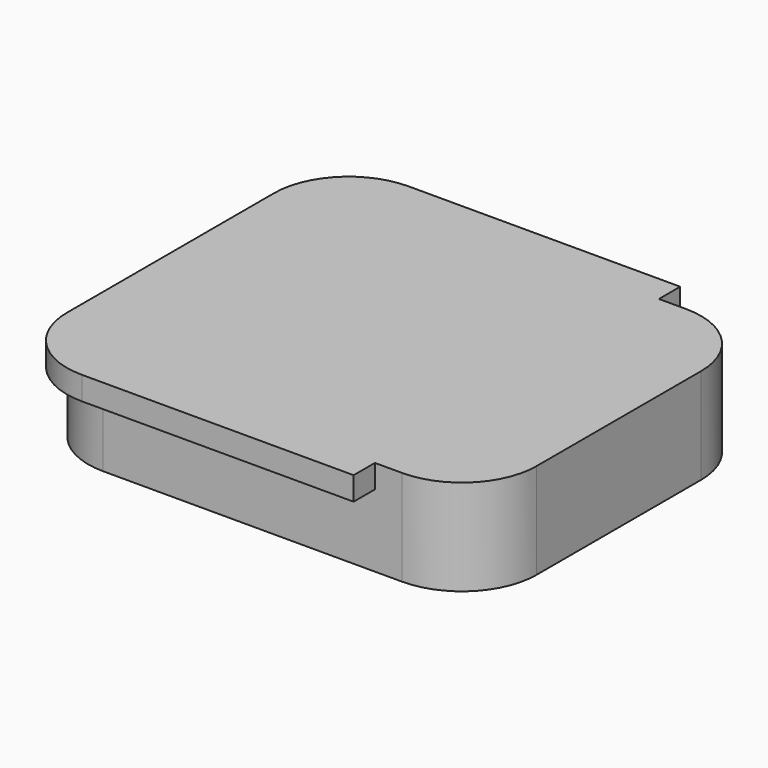
from build123d import *

# Parameters (mm, degrees)
F1_DEPTH     = 10.25
F3_DEPTH     = 2.5
F5_T         = 1.9
F5_T3_DEPTH  = 32.8875665362
F5_T5_DEPTH  = 6.3
F5_T8_ANGLE  = 90.000000001
F5_T10_ANGLE = 90.000000001


# Not quite as in the source:
# - a shell that OpenCascade refuses in one call is made with other operations: the cavity is built on its own and cut out


with BuildPart() as f1:
    # F0 (on Top) → F1 (new body)
    with BuildSketch(Plane.XY):
        with BuildLine():
            Line((14, 19), (-18, 19))
            ThreePointArc((-18, 19), (-23.6568542495, 16.6568542495), (-26, 11))
            Line((-26, 11), (-26, -11))
            ThreePointArc((-26, -11), (-23.6568542495, -16.6568542495), (-18, -19))
            Line((-18, -19), (14, -19))
            ThreePointArc((14, -19), (19.6568542495, -16.6568542495), (22, -11))
            Line((22, -11), (22, 11))
            ThreePointArc((22, 11), (19.6568542495, 16.6568542495), (14, 19))
        make_face()
    extrude(amount=F1_DEPTH)

    # F2 (on face) → F3 (join)
    with BuildSketch(Plane.XY.offset(10.25)):
        with BuildLine():
            Line((11.0875665362, 21.85), (-18, 21.85))
            ThreePointArc((-18, 21.85), (-23.6568542495, 19.5068542495), (-26, 13.85))
            Line((-26, 13.85), (-26, -13.85))
            ThreePointArc((-26, -13.85), (-23.6568542495, -19.5068542495), (-18, -21.85))
            Line((-18, -21.85), (11.0875665362, -21.85))
            Line((11.0875665362, -21.85), (11.0875665362, 21.85))
        make_face()
    extrude(amount=-F3_DEPTH)

    # F5: shell of thickness 1.9, made by hand


with BuildPart() as f5_core1:
    # F5_t2: copy of F1
    add(f1.part)

    # the walls: a layer under each face that stays
    f5_faces = [f5_core1.faces().sort_by_distance(p)[0] for p in [
        (-2, 19, 5.125),
        (19.6568542495, 16.6568542495, 5.125),
        (22, 0, 5.125),
        (19.6568542495, -16.6568542495, 5.125),
        (-2, -19, 5.125),
        (-23.6568542495, -16.6568542495, 3.875),
        (-26, 0, 5.125),
        (-23.6568542495, -19.5068542495, 9),
        (-3.4562167319, -21.85, 9),
        (-23.6568542495, 19.5068542495, 9),
        (-3.4562167319, 21.85, 9),
        (-19.8187389106, -20.0416666667, 7.75),
        (11.0875665362, -20.425, 9),
        (-2, 0, 10.25),
        (11.0875665362, 20.425, 9),
        (-19.8187389106, 20.0416666667, 7.75),
        (-23.6568542495, 16.6568542495, 3.875),
    ]]
    thicken(f5_faces, amount=-F5_T, mode=Mode.SUBTRACT)

    # F5_s4 → F5_t3 (cut)
    with BuildSketch(Plane.YZ.offset(-19.9)):
        Polygon((19.019, 7.731), (17.1, 7.75), (17.1, 9.65), (19, 9.65), align=None)
        Polygon((-19.019, 7.731), (-17.1, 7.75), (-17.1, 9.65), (-19, 9.65), align=None)
    extrude(amount=F5_T3_DEPTH, mode=Mode.SUBTRACT)

    # F5_s6 → F5_t5 (cut)
    with BuildSketch(Plane.XY.offset(5.85)):
        Polygon((11.1065665362, 19.019), (11.0875665362, 17.1), (9.1875665362, 17.1), (9.1875665362, 19), align=None)
        Polygon((11.1065665362, -19.019), (11.0875665362, -17.1), (9.1875665362, -17.1), (9.1875665362, -19), align=None)
    extrude(amount=F5_T5_DEPTH, mode=Mode.SUBTRACT)

    # F5_s7 → F5_t8 (revolve, cut)
    with BuildSketch(Plane.YZ.offset(-18)):
        Polygon((-19.019, 7.731), (-17.1, 7.75), (-17.1, 9.65), (-19, 9.65), align=None)
    revolve(axis=Axis((-18, -11, 7.75), (0, 0, -1)), revolution_arc=F5_T8_ANGLE, mode=Mode.SUBTRACT)

    # F5_s9 → F5_t10 (revolve, cut)
    with BuildSketch(Plane.XZ.offset(-11)):
        Polygon((-26.019, 7.731), (-26, 9.65), (-24.1, 9.65), (-24.1, 7.75), align=None)
    revolve(axis=Axis((-18, 11, 7.75), (0, 0, -1)), revolution_arc=F5_T10_ANGLE, mode=Mode.SUBTRACT)


with BuildPart() as f1_1:
    add(f1.part)

    # what is left inside the walls is the cavity
    f5_cavity = [f5_core1.part.solids().sort_by_distance(p)[0] for p in [
        (-2, -5.7, 0.019),
    ]]
    add(f5_cavity, mode=Mode.SUBTRACT)


solid = f1_1.part
